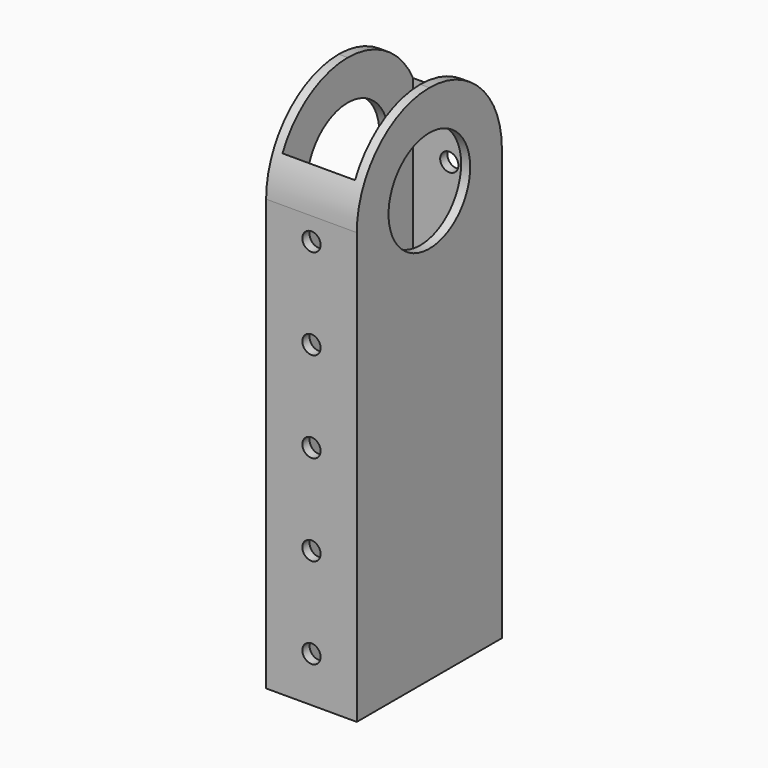
from build123d import *

# Parameters (mm, degrees)
F0_W     = 25.4
F0_H     = 50.8
F0_W_2   = 20.32
F0_H_2   = 45.72
F1_DEPTH = 146.05
F2_R     = 2.5527
F3_DEPTH = 76.2
F4_R     = 14.2875
F5_DEPTH = 25.4


# Not quite as in the source:
# - a feature names something its author has since deleted; it is built from what else it names


with BuildPart() as f1:
    # F0 (on Top) → F1 (new body)
    with BuildSketch(Plane.XY):
        with Locations((12.7, -25.4)):
            Rectangle(F0_W, F0_H)
        with Locations((12.7, -25.4)):
            Rectangle(F0_W_2, F0_H_2, mode=Mode.SUBTRACT)
    extrude(amount=F1_DEPTH)

    # F2 (on face) → F3 (cut)
    with BuildSketch(Plane.XZ.offset(50.8)):
        with Locations((12.7, 88.9)):
            Circle(F2_R)
        with Locations((12.7, 63.5)):
            Circle(F2_R)
        with Locations((12.7, 38.1)):
            Circle(F2_R)
        with Locations((12.7, 12.7)):
            Circle(F2_R)
        with Locations((12.7, 114.3)):
            Circle(F2_R)
        with Locations((12.7, 139.7)):
            Circle(F2_R)
    extrude(amount=-F3_DEPTH, mode=Mode.SUBTRACT)

    # F4 (on face) → F5 (cut)
    with BuildSketch(Plane.YZ.offset(25.4)):
        with Locations((-25.4, 120.65)):
            Circle(F4_R)
        with BuildLine():
            ThreePointArc((-50.8, 120.65), (-43.3605122421, 138.6105122421), (-25.4, 146.05))
            Line((-25.4, 146.05), (-50.8, 146.05))
            Line((-50.8, 146.05), (-50.8, 120.65))
        make_face()
        with BuildLine():
            ThreePointArc((-25.4, 146.05), (-7.4394877579, 138.6105122421), (0, 120.65))
            Line((0, 120.65), (0, 146.05))
            Line((0, 146.05), (-25.4, 146.05))
        make_face()
    extrude(amount=-F5_DEPTH, mode=Mode.SUBTRACT)


solid = f1.part
